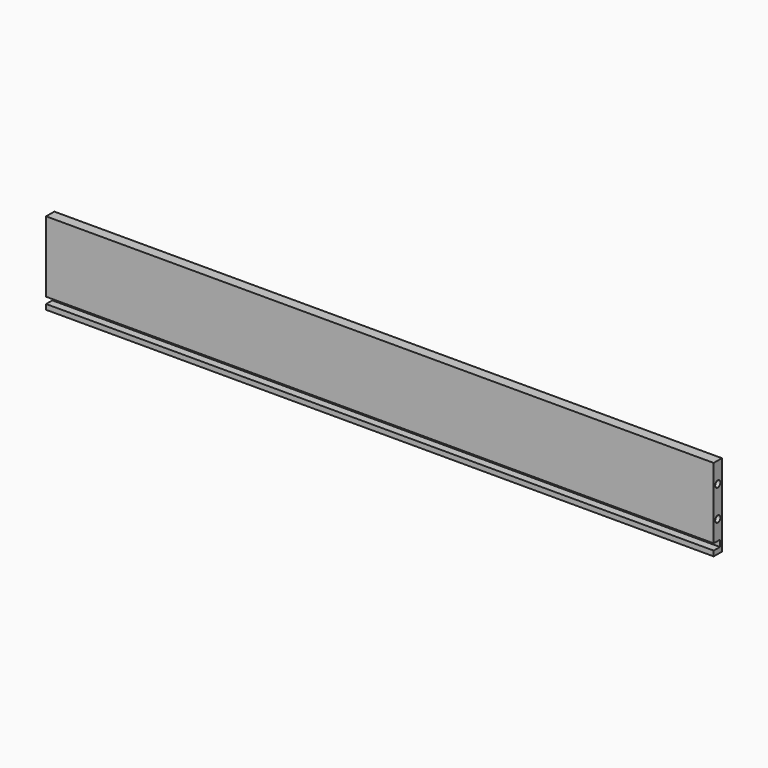
from build123d import *

# Parameters (mm, degrees)
F0_W     = 823.976
F0_H     = 101.6
F1_DEPTH = 12.7
F2_W     = 823.976
F2_H     = 7.874
F3_DEPTH = 9.652
F5_D     = 8.001
F5_DEPTH = 25.4
F5_TIP   = 2.4037429064
F7_D     = 8.001
F7_DEPTH = 25.4
F7_TIP   = 2.4037429064


# Not quite as in the source:
# - a feature names something its author has since deleted; it is built from what else it names


with BuildPart() as f1:
    # F0 (on Front) → F1 (new body)
    with BuildSketch(Plane.XZ):
        Rectangle(F0_W, F0_H)
    extrude(amount=F1_DEPTH)

    # F2 (on face) → F3 (cut)
    with BuildSketch(Plane.XZ.offset(12.7)):
        with Locations((0, -40.513)):
            Rectangle(F2_W, F2_H)
    extrude(amount=-F3_DEPTH, mode=Mode.SUBTRACT)

    # F5
    with Locations(Plane(origin=(-411.988, 0, 0), x_dir=(0, -1, 0), z_dir=(-1, 0, 0))):
        with Locations((6.35, 25.4), (6.35, -12.7)):
            Hole(F5_D / 2, depth=F5_DEPTH)
            with Locations((0, 0, -(F5_DEPTH + F5_TIP / 2))):  # 118° drill point
                Cone(0, F5_D / 2, F5_TIP, mode=Mode.SUBTRACT)

    # F7
    with Locations(Plane.YZ.offset(411.988)):
        with Locations((-6.35, 25.4), (-6.35, -12.7)):
            Hole(F7_D / 2, depth=F7_DEPTH)
            with Locations((0, 0, -(F7_DEPTH + F7_TIP / 2))):  # 118° drill point
                Cone(0, F7_D / 2, F7_TIP, mode=Mode.SUBTRACT)


solid = f1.part
